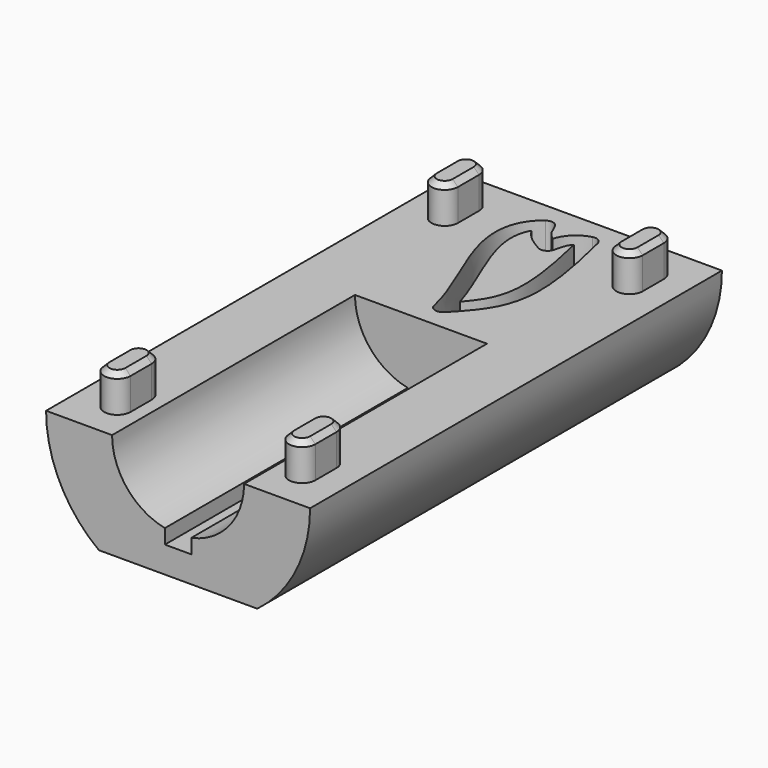
from build123d import *

# Parameters (mm, degrees)
F1_W      = 20
F1_H      = 39
F2_DEPTH  = 8
F4_DEPTH  = 23
F6_DEPTH  = 3
F8_W      = 2
F8_H      = 23
F9_DEPTH  = 6.0010001
F11_DEPTH = 39.0010001
F13_DEPTH = 2.8
F14_SIZE  = 0.4


# Not quite as in the source:
# - the dataset's text gives a spline's control points without its knots; the knots are read off the source's solid
# - a feature names something its author has since deleted; it is built from what else it names


with BuildPart() as f2:
    # F1 (on Top) → F2 (new body)
    with BuildSketch(Plane.XY):
        with Locations((0, 19.5)):
            Rectangle(F1_W, F1_H)
    extrude(amount=-F2_DEPTH)

    # F3 (on face) → F4 (cut)
    with BuildSketch(Plane.XZ):
        with BuildLine():
            ThreePointArc((-5, 0), (0, -5), (5, 0))
            Line((5, 0), (-5, 0))
        make_face()
    extrude(amount=-F4_DEPTH, mode=Mode.SUBTRACT)

    # F5 (on face) → F6 (cut)
    with BuildSketch(Plane.XY):
        with BuildLine():
            ThreePointArc((-2.3557534961, 36.7738627595), (-2.3769706924, 37.1646354158), (-2.1527294294, 37.4853678498))
            add(Edge.make_bspline(
                [(-2.1527294294, 37.4853678498), (-2.5671901237, 37.1841684929), (-3.055117682, 36.6166735378), (-3.4122374969, 35.7157419772), (-3.5912952772, 34.750955586), (-3.5372299448, 33.7149471429), (-3.3000662924, 32.6256335644), (-2.9634860661, 31.5141507712), (-2.4061383857, 30.0818122717), (-1.4054540892, 27.7353813397), (-0.7372439498, 25.9732231452), (-0.5002933365, 24.8736098595)],
                knots=[0, 0, 0, 0, 0.125, 0.1875, 0.25, 0.375, 0.4375, 0.5, 0.625, 0.75, 1, 1, 1, 1], degree=3))
            ThreePointArc((-0.5002933365, 24.8736098595), (-0.4909168058, 25.1639692369), (-0.3462338651, 25.4158885376))
            add(Edge.make_bspline(
                [(-0.0845567639, 25.6909345906), (-0.167834195, 25.6023614379), (-0.254995182, 25.5107665333), (-0.3462338651, 25.4158885376)],
                knots=[0.9719318269, 0.9719318269, 0.9719318269, 0.9719318269, 1, 1, 1, 1], degree=3))
            add(Edge.make_bspline(
                [(-2.2699116487, 36.5680125793), (-2.9682117374, 35.7518079098), (-3.2999864497, 32.664782733), (-0.8006894411, 28.2786821734), (-0.0845567639, 25.6909345906)],
                knots=[0.0649424521, 0.0649424521, 0.0649424521, 0.0649424521, 0.4011494105, 0.9508193746, 0.9508193746, 0.9508193746, 0.9508193746], degree=3))
            add(Edge.make_bspline(
                [(-2.3557534961, 36.7738627595), (-2.3261190111, 36.7010332307), (-2.2975533288, 36.6325615414), (-2.2699116487, 36.5680125793)],
                knots=[0, 0, 0, 0, 0.042291898, 0.042291898, 0.042291898, 0.042291898], degree=3))
        make_face()
        with BuildLine():
            add(Edge.make_bspline(
                [(-1.8, 37), (-1.9787847666, 36.8700724641), (-2.1350265165, 36.7256724113), (-2.2699116487, 36.5680125793)],
                knots=[0, 0, 0, 0, 0.0649424521, 0.0649424521, 0.0649424521, 0.0649424521], degree=3))
            add(Edge.make_bspline(
                [(-1.8, 37), (-1.7042391513, 36.7646587251), (-1.6219968428, 36.5816224105), (-1.549515289, 36.4360042756)],
                knots=[0, 0, 0, 0, 0.1427519756, 0.1427519756, 0.1427519756, 0.1427519756], degree=3))
            add(Edge.make_bspline(
                [(-1.4472705706, 36.5146321502), (-1.482632785, 36.48893351), (-1.5166959819, 36.4627326553), (-1.549515289, 36.4360042756)],
                knots=[0, 0, 0, 0, 0.0161452213, 0.0161452213, 0.0161452213, 0.0161452213], degree=3))
            ThreePointArc((-1.4472705706, 36.5146321502), (-1.2230293076, 36.8353645842), (-1.2442465039, 37.2261372405))
            ThreePointArc((-1.2442465039, 37.2261372405), (-1.6353645842, 37.5769706924), (-2.1527294294, 37.4853678498))
            ThreePointArc((-2.1527294294, 37.4853678498), (-2.3769706924, 37.1646354158), (-2.3557534961, 36.7738627595))
            add(Edge.make_bspline(
                [(-2.3557534961, 36.7738627595), (-2.3261190111, 36.7010332307), (-2.2975533288, 36.6325615414), (-2.2699116487, 36.5680125793)],
                knots=[0, 0, 0, 0, 0.042291898, 0.042291898, 0.042291898, 0.042291898], degree=3))
        make_face()
        with BuildLine():
            add(Edge.make_bspline(
                [(-1.8, 37), (-1.7042391513, 36.7646587251), (-1.6219968428, 36.5816224105), (-1.549515289, 36.4360042756)],
                knots=[0, 0, 0, 0, 0.1427519756, 0.1427519756, 0.1427519756, 0.1427519756], degree=3))
            add(Edge.make_bspline(
                [(-1.8, 37), (-1.9787847666, 36.8700724641), (-2.1350265165, 36.7256724113), (-2.2699116487, 36.5680125793)],
                knots=[0, 0, 0, 0, 0.0649424521, 0.0649424521, 0.0649424521, 0.0649424521], degree=3))
            add(Edge.make_bspline(
                [(-2.2699116487, 36.5680125793), (-2.2158542286, 36.4417774752), (-2.1136998623, 36.2168747945), (-2.0215650079, 36.0400008797), (-1.9764958817, 35.9600370034)],
                knots=[0.042291898, 0.042291898, 0.042291898, 0.042291898, 0.125, 0.2095208321, 0.2095208321, 0.2095208321, 0.2095208321], degree=3))
            add(Edge.make_bspline(
                [(-1.549515289, 36.4360042756), (-1.7243723299, 36.2935989117), (-1.8639200522, 36.1362191151), (-1.9764958817, 35.9600370034)],
                knots=[0.0161452213, 0.0161452213, 0.0161452213, 0.0161452213, 0.1021648807, 0.1021648807, 0.1021648807, 0.1021648807], degree=3))
        make_face()
        with BuildLine():
            add(Edge.make_bspline(
                [(-2.2699116487, 36.5680125793), (-2.2158542286, 36.4417774752), (-2.1136998623, 36.2168747945), (-2.0215650079, 36.0400008797), (-1.9764958817, 35.9600370034)],
                knots=[0.042291898, 0.042291898, 0.042291898, 0.042291898, 0.125, 0.2095208321, 0.2095208321, 0.2095208321, 0.2095208321], degree=3))
            add(Edge.make_bspline(
                [(-2.2699116487, 36.5680125793), (-2.9682117374, 35.7518079098), (-3.2999864497, 32.664782733), (-0.8006894411, 28.2786821734), (-0.0845567639, 25.6909345906)],
                knots=[0.0649424521, 0.0649424521, 0.0649424521, 0.0649424521, 0.4011494105, 0.9508193746, 0.9508193746, 0.9508193746, 0.9508193746], degree=3))
            add(Edge.make_bspline(
                [(0.3895721523, 26.2103233244), (0.247389863, 26.0488583662), (0.0899422675, 25.8765302454), (-0.0845567639, 25.6909345906)],
                knots=[0.9131179447, 0.9131179447, 0.9131179447, 0.9131179447, 0.9719318269, 0.9719318269, 0.9719318269, 0.9719318269], degree=3))
            add(Edge.make_bspline(
                [(-1.9764958817, 35.9600370034), (-2.0063807071, 35.9132670026), (-2.1109575779, 35.733535323), (-2.2499152092, 35.3883775969), (-2.3795057258, 34.7059753565), (-2.3435032802, 33.8767933474), (-2.139298662, 32.9350788197), (-1.8332292669, 31.9209391633), (-1.2995768366, 30.5463194368), (-0.5501596185, 28.7880925237), (0.0294188469, 27.3260478108), (0.3132731916, 26.4623723407), (0.3895721523, 26.2103233244)],
                knots=[0.1021648807, 0.1021648807, 0.1021648807, 0.1021648807, 0.125, 0.1875, 0.25, 0.375, 0.4375, 0.5, 0.625, 0.75, 0.875, 0.9264050525, 0.9264050525, 0.9264050525, 0.9264050525], degree=3))
        make_face()
        with BuildLine():
            add(Edge.make_bspline(
                [(-0.5398704721, 35.3252999862), (-0.4996637471, 35.4953294599), (-0.4501302625, 35.6958108337), (-0.3837930151, 35.8979652695), (-0.3706897734, 35.9357783226)],
                knots=[0.0663486573, 0.0663486573, 0.0663486573, 0.0663486573, 0.25, 0.2922049943, 0.2922049943, 0.2922049943, 0.2922049943], degree=3))
            add(Edge.make_bspline(
                [(-0.5398704523, 35.3252999871), (-0.4010210547, 35.2348626653), (-0.2258354649, 35.1285546076), (0, 35)],
                knots=[0.8589437324, 0.8589437324, 0.8589437324, 0.8589437324, 1, 1, 1, 1], degree=3))
            add(Edge.make_bspline(
                [(0, 35), (0.0532776461, 35.2256223212), (0.0985342253, 35.4231853411), (0.1527780376, 35.6044457963)],
                knots=[0, 0, 0, 0, 0.2328464411, 0.2328464411, 0.2328464411, 0.2328464411], degree=3))
            add(Edge.make_bspline(
                [(-0.3706897734, 35.9357783226), (-0.3161533695, 35.896700895), (-0.1780179648, 35.8030089583), (0.0258347324, 35.6785715207), (0.1527780376, 35.6044457963)],
                knots=[0.7894774807, 0.7894774807, 0.7894774807, 0.7894774807, 0.875, 0.9671443967, 0.9671443967, 0.9671443967, 0.9671443967], degree=3))
        make_face()
        with BuildLine():
            add(Edge.make_bspline(
                [(-0.5398704523, 35.3252999871), (-0.4010210547, 35.2348626653), (-0.2258354649, 35.1285546076), (0, 35)],
                knots=[0.8589437324, 0.8589437324, 0.8589437324, 0.8589437324, 1, 1, 1, 1], degree=3))
            add(Edge.make_bspline(
                [(-0.5839404564, 35.137889606), (-0.5689126336, 35.2015300349), (-0.5543961608, 35.263872571), (-0.5398704721, 35.3252999862)],
                knots=[0, 0, 0, 0, 0.0663486573, 0.0663486573, 0.0663486573, 0.0663486573], degree=3))
            ThreePointArc((-0.5839404564, 35.137889606), (-0.5501033986, 34.7604457247), (-0.2968227148, 34.4785632579))
            ThreePointArc((-0.2968227148, 34.4785632579), (0.2395542753, 34.4498966014), (0.5839404564, 34.862110394))
            ThreePointArc((0.5839404564, 34.862110394), (0.5501033986, 35.2395542753), (0.2968227148, 35.5214367421))
            add(Edge.make_bspline(
                [(0.1527780376, 35.6044457963), (0.1980417652, 35.5780150477), (0.2460031457, 35.5503652798), (0.2968227148, 35.5214367421)],
                knots=[0.9671443967, 0.9671443967, 0.9671443967, 0.9671443967, 1, 1, 1, 1], degree=3))
            add(Edge.make_bspline(
                [(0, 35), (0.0532776461, 35.2256223212), (0.0985342253, 35.4231853411), (0.1527780376, 35.6044457963)],
                knots=[0, 0, 0, 0, 0.2328464411, 0.2328464411, 0.2328464411, 0.2328464411], degree=3))
        make_face()
        with BuildLine():
            add(Edge.make_bspline(
                [(0.5839404564, 34.862110394), (0.641721126, 35.1068023006), (0.7112742607, 35.4046889034), (0.814148382, 35.6879713765), (0.9077943888, 35.8708676461), (1.0072594782, 36.0093722861), (1.0764543119, 36.0834718482), (1.0981810502, 36.1049356243)],
                knots=[0, 0, 0, 0, 0.25, 0.375, 0.5, 0.625, 0.6780239279, 0.6780239279, 0.6780239279, 0.6780239279], degree=3))
            add(Edge.make_bspline(
                [(0.9438460932, 36.7485646305), (0.9976399468, 36.5282774215), (1.0490628639, 36.313797947), (1.0981810502, 36.1049356243)],
                knots=[0.0040855324, 0.0040855324, 0.0040855324, 0.0040855324, 0.0291170539, 0.0291170539, 0.0291170539, 0.0291170539], degree=3))
            add(Edge.make_bspline(
                [(0.1527780376, 35.6044457963), (0.2101663079, 35.7962137339), (0.3665971644, 36.1986585161), (0.6854791516, 36.5778369652), (0.9438460932, 36.7485646305)],
                knots=[0.2328464411, 0.2328464411, 0.2328464411, 0.2328464411, 0.4791907511, 0.8041909219, 0.8041909219, 0.8041909219, 0.8041909219], degree=3))
            add(Edge.make_bspline(
                [(0.1527780376, 35.6044457963), (0.1980417652, 35.5780150477), (0.2460031457, 35.5503652798), (0.2968227148, 35.5214367421)],
                knots=[0.9671443967, 0.9671443967, 0.9671443967, 0.9671443967, 1, 1, 1, 1], degree=3))
            ThreePointArc((0.2968227148, 35.5214367421), (0.5501033986, 35.2395542753), (0.5839404564, 34.862110394))
        make_face()
        with BuildLine():
            add(Edge.make_bspline(
                [(-0.3706897734, 35.9357783226), (-0.3061763614, 36.1219497391), (-0.1754059358, 36.4215556963), (0.1155960329, 36.827916004), (0.5407139223, 37.2419464227), (0.9868880869, 37.4773003712), (1.3350055159, 37.5768681134)],
                knots=[0.2922049943, 0.2922049943, 0.2922049943, 0.2922049943, 0.5, 0.625, 0.75, 1, 1, 1, 1], degree=3))
            add(Edge.make_bspline(
                [(-0.3706897734, 35.9357783226), (-0.3161533695, 35.896700895), (-0.1780179648, 35.8030089583), (0.0258347324, 35.6785715207), (0.1527780376, 35.6044457963)],
                knots=[0.7894774807, 0.7894774807, 0.7894774807, 0.7894774807, 0.875, 0.9671443967, 0.9671443967, 0.9671443967, 0.9671443967], degree=3))
            add(Edge.make_bspline(
                [(0.1527780376, 35.6044457963), (0.2101663079, 35.7962137339), (0.3665971644, 36.1986585161), (0.6854791516, 36.5778369652), (0.9438460932, 36.7485646305)],
                knots=[0.2328464411, 0.2328464411, 0.2328464411, 0.2328464411, 0.4791907511, 0.8041909219, 0.8041909219, 0.8041909219, 0.8041909219], degree=3))
            add(Edge.make_bspline(
                [(0.9173163523, 36.8568924647), (0.9262229513, 36.8206279202), (0.9350661023, 36.7845189183), (0.9438460932, 36.7485646305)],
                knots=[0, 0, 0, 0, 0.0040855324, 0.0040855324, 0.0040855324, 0.0040855324], degree=3))
            ThreePointArc((0.9173163523, 36.8568924647), (0.9810136024, 37.3010865642), (1.3350055159, 37.5768681134))
        make_face()
        with BuildLine():
            ThreePointArc((2.0826836477, 37.1431075353), (1.8010865642, 37.5189863976), (1.3350055159, 37.5768681134))
            ThreePointArc((1.3350055159, 37.5768681134), (0.9810136024, 37.3010865642), (0.9173163523, 36.8568924647))
            add(Edge.make_bspline(
                [(0.9173163523, 36.8568924647), (0.9262229513, 36.8206279202), (0.9350661023, 36.7845189183), (0.9438460932, 36.7485646305)],
                knots=[0, 0, 0, 0, 0.0040855324, 0.0040855324, 0.0040855324, 0.0040855324], degree=3))
            add(Edge.make_bspline(
                [(0.9438460932, 36.7485646305), (1.0995093734, 36.8514261972), (1.2831144249, 36.9379668892), (1.5, 37)],
                knots=[0.8041909219, 0.8041909219, 0.8041909219, 0.8041909219, 1, 1, 1, 1], degree=3))
            add(Edge.make_bspline(
                [(1.5, 37), (1.5489102697, 36.800854551), (1.5959430164, 36.6062788827), (1.6411443659, 36.4161321311)],
                knots=[0, 0, 0, 0, 0.0222790414, 0.0222790414, 0.0222790414, 0.0222790414], degree=3))
            add(Edge.make_bspline(
                [(1.6411443659, 36.4161321311), (1.6490072659, 36.4184994954), (1.6569567473, 36.4208329517), (1.6649944841, 36.4231318866)],
                knots=[0.9902313132, 0.9902313132, 0.9902313132, 0.9902313132, 1, 1, 1, 1], degree=3))
            ThreePointArc((1.6649944841, 36.4231318866), (2.0189863976, 36.6989134358), (2.0826836477, 37.1431075353))
        make_face()
        with BuildLine():
            add(Edge.make_bspline(
                [(0.9438460932, 36.7485646305), (0.9976399468, 36.5282774215), (1.0490628639, 36.313797947), (1.0981810502, 36.1049356243)],
                knots=[0.0040855324, 0.0040855324, 0.0040855324, 0.0040855324, 0.0291170539, 0.0291170539, 0.0291170539, 0.0291170539], degree=3))
            add(Edge.make_bspline(
                [(1.0981810502, 36.1049356243), (1.1276734955, 36.1340711176), (1.2645312847, 36.2556027708), (1.4477801167, 36.3579139666), (1.6411443659, 36.4161321311)],
                knots=[0.6780239279, 0.6780239279, 0.6780239279, 0.6780239279, 0.75, 0.9902313132, 0.9902313132, 0.9902313132, 0.9902313132], degree=3))
            add(Edge.make_bspline(
                [(1.5, 37), (1.5489102697, 36.800854551), (1.5959430164, 36.6062788827), (1.6411443659, 36.4161321311)],
                knots=[0, 0, 0, 0, 0.0222790414, 0.0222790414, 0.0222790414, 0.0222790414], degree=3))
            add(Edge.make_bspline(
                [(0.9438460932, 36.7485646305), (1.0995093734, 36.8514261972), (1.2831144249, 36.9379668892), (1.5, 37)],
                knots=[0.8041909219, 0.8041909219, 0.8041909219, 0.8041909219, 1, 1, 1, 1], degree=3))
        make_face()
        with BuildLine():
            add(Edge.make_bspline(
                [(1.0981810502, 36.1049356243), (1.2863276802, 35.3048909754), (1.6418538615, 33.6517149147), (1.9484782003, 31.6588848612), (2.0263224122, 30.0903506861), (1.9295867934, 29.1561038885), (1.7844118929, 28.5453007445), (1.6444967664, 28.1249387584), (1.4799522014, 27.7395563792), (1.2059996187, 27.2366555132), (0.8486194347, 26.7432605343), (0.4817221082, 26.314970597), (0.3895721523, 26.2103233244)],
                knots=[0.0291170539, 0.0291170539, 0.0291170539, 0.0291170539, 0.125, 0.25, 0.375, 0.5, 0.5625, 0.625, 0.6875, 0.75, 0.875, 0.9131179447, 0.9131179447, 0.9131179447, 0.9131179447], degree=3))
            add(Edge.make_bspline(
                [(0.3895721523, 26.2103233244), (0.4586961228, 25.9819764558), (0.5225530701, 25.7533251253), (0.5798667503, 25.5245971385)],
                knots=[0.9264050525, 0.9264050525, 0.9264050525, 0.9264050525, 0.9729760843, 0.9729760843, 0.9729760843, 0.9729760843], degree=3))
            add(Edge.make_bspline(
                [(1.6411443659, 36.4161321311), (2.8299076099, 31.4154082186), (2.7070712048, 28.361405173), (1.5216174051, 26.5521371181), (0.5798667503, 25.5245971385)],
                knots=[0.0222790414, 0.0222790414, 0.0222790414, 0.0222790414, 0.6082019369, 0.9458681718, 0.9458681718, 0.9458681718, 0.9458681718], degree=3))
            add(Edge.make_bspline(
                [(1.0981810502, 36.1049356243), (1.1276734955, 36.1340711176), (1.2645312847, 36.2556027708), (1.4477801167, 36.3579139666), (1.6411443659, 36.4161321311)],
                knots=[0.6780239279, 0.6780239279, 0.6780239279, 0.6780239279, 0.75, 0.9902313132, 0.9902313132, 0.9902313132, 0.9902313132], degree=3))
        make_face()
        with BuildLine():
            add(Edge.make_bspline(
                [(1.6411443659, 36.4161321311), (2.8299076099, 31.4154082186), (2.7070712048, 28.361405173), (1.5216174051, 26.5521371181), (0.5798667503, 25.5245971385)],
                knots=[0.0222790414, 0.0222790414, 0.0222790414, 0.0222790414, 0.6082019369, 0.9458681718, 0.9458681718, 0.9458681718, 0.9458681718], degree=3))
            add(Edge.make_bspline(
                [(0.5798667503, 25.5245971385), (0.6131243356, 25.3918724471), (0.6441786926, 25.2591219443), (0.672780459, 25.1263901405)],
                knots=[0.9729760843, 0.9729760843, 0.9729760843, 0.9729760843, 1, 1, 1, 1], degree=3))
            ThreePointArc((0.672780459, 25.1263901405), (0.6634039283, 24.8360307631), (0.5187209876, 24.5841114624))
            add(Edge.make_bspline(
                [(2.0826836477, 37.1431075353), (2.3590166471, 36.0179765654), (2.7940502318, 34.0519174423), (3.1420540935, 31.7993404764), (3.2160092922, 30.3696505967), (3.164403491, 29.4177296717), (3.0749202627, 28.7837597633), (2.9395048641, 28.2146521567), (2.7695695652, 27.7035891202), (2.5615536726, 27.2153231179), (2.2126370827, 26.5759259812), (1.6253506034, 25.7726740804), (0.9372865117, 25.0193726545), (0.5187209876, 24.5841114624)],
                knots=[0, 0, 0, 0, 0.125, 0.25, 0.375, 0.4375, 0.5, 0.5625, 0.625, 0.6875, 0.75, 0.875, 1, 1, 1, 1], degree=3))
            ThreePointArc((2.0826836477, 37.1431075353), (2.0189863976, 36.6989134358), (1.6649944841, 36.4231318866))
            add(Edge.make_bspline(
                [(1.6411443659, 36.4161321311), (1.6490072659, 36.4184994954), (1.6569567473, 36.4208329517), (1.6649944841, 36.4231318866)],
                knots=[0.9902313132, 0.9902313132, 0.9902313132, 0.9902313132, 1, 1, 1, 1], degree=3))
        make_face()
        with BuildLine():
            add(Edge.make_bspline(
                [(0.3895721523, 26.2103233244), (0.247389863, 26.0488583662), (0.0899422675, 25.8765302454), (-0.0845567639, 25.6909345906)],
                knots=[0.9131179447, 0.9131179447, 0.9131179447, 0.9131179447, 0.9719318269, 0.9719318269, 0.9719318269, 0.9719318269], degree=3))
            add(Edge.make_bspline(
                [(-0.0845567639, 25.6909345906), (-0.0204822188, 25.4594010291), (0.0369107304, 25.2289381548), (0.0862435612, 25)],
                knots=[0.9508193746, 0.9508193746, 0.9508193746, 0.9508193746, 1, 1, 1, 1], degree=3))
            add(Edge.make_bspline(
                [(0.5798667503, 25.5245971385), (0.4288931574, 25.3598705181), (0.2648551596, 25.1857360264), (0.0862435612, 25)],
                knots=[0.9458681718, 0.9458681718, 0.9458681718, 0.9458681718, 1, 1, 1, 1], degree=3))
            add(Edge.make_bspline(
                [(0.3895721523, 26.2103233244), (0.4586961228, 25.9819764558), (0.5225530701, 25.7533251253), (0.5798667503, 25.5245971385)],
                knots=[0.9264050525, 0.9264050525, 0.9264050525, 0.9264050525, 0.9729760843, 0.9729760843, 0.9729760843, 0.9729760843], degree=3))
        make_face()
        with BuildLine():
            add(Edge.make_bspline(
                [(-0.0845567639, 25.6909345906), (-0.0204822188, 25.4594010291), (0.0369107304, 25.2289381548), (0.0862435612, 25)],
                knots=[0.9508193746, 0.9508193746, 0.9508193746, 0.9508193746, 1, 1, 1, 1], degree=3))
            add(Edge.make_bspline(
                [(-0.0845567639, 25.6909345906), (-0.167834195, 25.6023614379), (-0.254995182, 25.5107665333), (-0.3462338651, 25.4158885376)],
                knots=[0.9719318269, 0.9719318269, 0.9719318269, 0.9719318269, 1, 1, 1, 1], degree=3))
            ThreePointArc((-0.3462338651, 25.4158885376), (-0.4909168058, 25.1639692369), (-0.5002933365, 24.8736098595))
            ThreePointArc((-0.5002933365, 24.8736098595), (-0.0777256757, 24.4228396329), (0.5187209876, 24.5841114624))
            ThreePointArc((0.5187209876, 24.5841114624), (0.6634039283, 24.8360307631), (0.672780459, 25.1263901405))
            add(Edge.make_bspline(
                [(0.5798667503, 25.5245971385), (0.6131243356, 25.3918724471), (0.6441786926, 25.2591219443), (0.672780459, 25.1263901405)],
                knots=[0.9729760843, 0.9729760843, 0.9729760843, 0.9729760843, 1, 1, 1, 1], degree=3))
            add(Edge.make_bspline(
                [(0.5798667503, 25.5245971385), (0.4288931574, 25.3598705181), (0.2648551596, 25.1857360264), (0.0862435612, 25)],
                knots=[0.9458681718, 0.9458681718, 0.9458681718, 0.9458681718, 1, 1, 1, 1], degree=3))
        make_face()
        with BuildLine():
            add(Edge.make_bspline(
                [(-1.549515289, 36.4360042756), (-1.3698705044, 36.0750912281), (-1.127599738, 35.8098026143), (-0.8965833191, 35.5576391754), (-0.5398704523, 35.3252999871)],
                knots=[0.1427519756, 0.1427519756, 0.1427519756, 0.1427519756, 0.4965612771, 0.8589437324, 0.8589437324, 0.8589437324, 0.8589437324], degree=3))
            add(Edge.make_bspline(
                [(-1.549515289, 36.4360042756), (-1.7243723299, 36.2935989117), (-1.8639200522, 36.1362191151), (-1.9764958817, 35.9600370034)],
                knots=[0.0161452213, 0.0161452213, 0.0161452213, 0.0161452213, 0.1021648807, 0.1021648807, 0.1021648807, 0.1021648807], degree=3))
            add(Edge.make_bspline(
                [(-1.9764958817, 35.9600370034), (-1.9549111353, 35.9217402771), (-1.9008733645, 35.829816818), (-1.8163985518, 35.7013605906), (-1.7240586275, 35.5793219123), (-1.6538235442, 35.4971848798), (-1.6043222887, 35.4421937331), (-1.5623968339, 35.3963885038), (-1.5050727097, 35.3337169676), (-1.4148399703, 35.2417924069), (-1.3044546138, 35.1412725211), (-1.1275440778, 34.998196209), (-0.8412029644, 34.7990514743), (-0.5037361019, 34.5963466597), (-0.2968227148, 34.4785632579)],
                knots=[0.2095208321, 0.2095208321, 0.2095208321, 0.2095208321, 0.25, 0.3125, 0.375, 0.4375, 0.46875, 0.5, 0.5625, 0.625, 0.6875, 0.75, 0.875, 1, 1, 1, 1], degree=3))
            ThreePointArc((-0.2968227148, 34.4785632579), (-0.5501033986, 34.7604457247), (-0.5839404564, 35.137889606))
            add(Edge.make_bspline(
                [(-0.5839404564, 35.137889606), (-0.5689126336, 35.2015300349), (-0.5543961608, 35.263872571), (-0.5398704721, 35.3252999862)],
                knots=[0, 0, 0, 0, 0.0663486573, 0.0663486573, 0.0663486573, 0.0663486573], degree=3))
        make_face()
        with BuildLine():
            add(Edge.make_bspline(
                [(-1.4472705706, 36.5146321502), (-1.482632785, 36.48893351), (-1.5166959819, 36.4627326553), (-1.549515289, 36.4360042756)],
                knots=[0, 0, 0, 0, 0.0161452213, 0.0161452213, 0.0161452213, 0.0161452213], degree=3))
            add(Edge.make_bspline(
                [(-1.549515289, 36.4360042756), (-1.3698705044, 36.0750912281), (-1.127599738, 35.8098026143), (-0.8965833191, 35.5576391754), (-0.5398704523, 35.3252999871)],
                knots=[0.1427519756, 0.1427519756, 0.1427519756, 0.1427519756, 0.4965612771, 0.8589437324, 0.8589437324, 0.8589437324, 0.8589437324], degree=3))
            add(Edge.make_bspline(
                [(-0.5398704721, 35.3252999862), (-0.4996637471, 35.4953294599), (-0.4501302625, 35.6958108337), (-0.3837930151, 35.8979652695), (-0.3706897734, 35.9357783226)],
                knots=[0.0663486573, 0.0663486573, 0.0663486573, 0.0663486573, 0.25, 0.2922049943, 0.2922049943, 0.2922049943, 0.2922049943], degree=3))
            add(Edge.make_bspline(
                [(-1.2442465039, 37.2261372405), (-1.1641306911, 37.02924511), (-1.0266868462, 36.7197419028), (-0.9053150564, 36.4997887495), (-0.8336442487, 36.3915436939), (-0.7886871867, 36.3322016326), (-0.7515038411, 36.2884842927), (-0.7173622243, 36.2504833644), (-0.6765872722, 36.2058915248), (-0.6307698593, 36.1560090966), (-0.5824526351, 36.1070803181), (-0.5246233931, 36.0542601816), (-0.4543120612, 35.9970978044), (-0.3958639597, 35.9538165938), (-0.3706897734, 35.9357783226)],
                knots=[0, 0, 0, 0, 0.125, 0.25, 0.3125, 0.375, 0.4375, 0.46875, 0.5, 0.5625, 0.625, 0.6875, 0.75, 0.7894774807, 0.7894774807, 0.7894774807, 0.7894774807], degree=3))
            ThreePointArc((-1.2442465039, 37.2261372405), (-1.2230293076, 36.8353645842), (-1.4472705706, 36.5146321502))
        make_face()
    extrude(amount=-F6_DEPTH, mode=Mode.SUBTRACT)

    # F8 (on offset) → F9 (cut, through all)
    with BuildSketch(Plane.XY.offset(-6)):
        with Locations((0, 11.5)):
            Rectangle(F8_W, F8_H)
    extrude(amount=F9_DEPTH, mode=Mode.SUBTRACT)

    # F10 (on face) → F11 (cut, through all)
    with BuildSketch(Plane.XZ):
        with BuildLine():
            ThreePointArc((-6, -8), (-8.94427191, -4.472135955), (-10, 0))
            Line((-10, 0), (-10, -8))
            Line((-10, -8), (-6, -8))
        make_face()
        with BuildLine():
            Line((10, -8), (10, 0))
            ThreePointArc((10, 0), (8.94427191, -4.472135955), (6, -8))
            Line((6, -8), (10, -8))
        make_face()
    extrude(amount=-F11_DEPTH, mode=Mode.SUBTRACT)

    # F12 (on face) → F13 (join)
    with BuildSketch(Plane.XY):
        with BuildLine():
            ThreePointArc((-6, 5), (-7, 6), (-8, 5))
            Line((-8, 5), (-8, 3))
            ThreePointArc((-8, 3), (-7, 2), (-6, 3))
            Line((-6, 3), (-6, 5))
        make_face()
        with BuildLine():
            ThreePointArc((8, 5), (7, 6), (6, 5))
            Line((6, 5), (6, 3))
            ThreePointArc((6, 3), (7, 2), (8, 3))
            Line((8, 3), (8, 5))
        make_face()
        with BuildLine():
            ThreePointArc((-6, 36), (-7, 37), (-8, 36))
            Line((-8, 36), (-8, 34))
            ThreePointArc((-8, 34), (-7, 33), (-6, 34))
            Line((-6, 34), (-6, 36))
        make_face()
        with BuildLine():
            ThreePointArc((8, 36), (7, 37), (6, 36))
            Line((6, 36), (6, 34))
            ThreePointArc((6, 34), (7, 33), (8, 34))
            Line((8, 34), (8, 36))
        make_face()
    extrude(amount=F13_DEPTH)

    # F14
    f14_edges = [f2.edges().sort_by_distance(p)[0] for p in [
        (-7, 6, 2.8),
        (-8, 4, 2.8),
        (-7, 2, 2.8),
        (-6, 4, 2.8),
        (7, 6, 2.8),
        (6, 4, 2.8),
        (7, 2, 2.8),
        (8, 4, 2.8),
        (-7, 37, 2.8),
        (-8, 35, 2.8),
        (-7, 33, 2.8),
        (-6, 35, 2.8),
        (7, 37, 2.8),
        (6, 35, 2.8),
        (7, 33, 2.8),
        (8, 35, 2.8),
    ]]
    chamfer(f14_edges, length=F14_SIZE)


solid = f2.part
